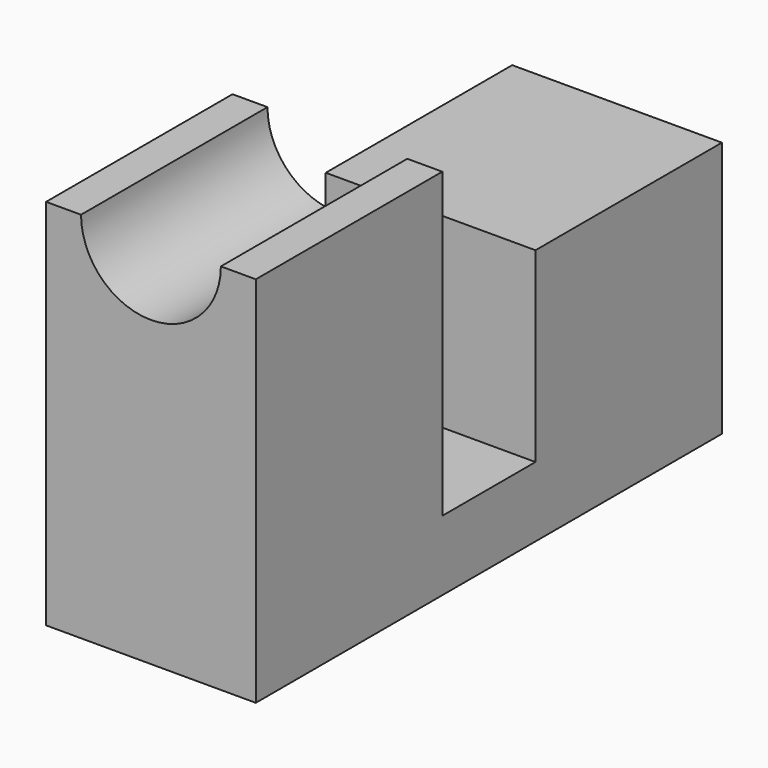
from build123d import *

# Parameters (mm, degrees)
F0_W     = 9
F0_H     = 10
F1_DEPTH = 13
F3_DEPTH = 25
F4_W     = 9
F4_H     = 10
F4_H_2   = 15
F5_DEPTH = 3
F6_W     = 9
F6_H     = 10
F7_DEPTH = 8


# Not quite as in the source:
# - a feature names something its author has since deleted; it is built from what else it names


with BuildPart() as f1:
    # F0 (on Top) → F1 (new body)
    with BuildSketch(Plane.XY):
        with Locations((4.5, 5)):
            Rectangle(F0_W, F0_H)
    extrude(amount=F1_DEPTH)

    # F2 (on face) → F3 (cut)
    with BuildSketch(Plane.XZ):
        with BuildLine():
            ThreePointArc((1.5, 13), (4.5, 10), (7.5, 13))
            Line((7.5, 13), (1.5, 13))
        make_face()
    extrude(amount=-F3_DEPTH, mode=Mode.SUBTRACT)

    # F4 (on face) → F5 (join)
    with BuildSketch(Plane(origin=(0, 0, 0), x_dir=(1, 0, 0), z_dir=(0, 0, -1))):
        with Locations((4.5, -5)):
            Rectangle(F4_W, F4_H)
        with Locations((4.5, -17.5)):
            Rectangle(F4_W, F4_H_2)
    extrude(amount=F5_DEPTH)

    # F6 (on face) → F7 (join)
    with BuildSketch(Plane.XY):
        with Locations((4.5, 20)):
            Rectangle(F6_W, F6_H)
    extrude(amount=F7_DEPTH)


solid = f1.part
